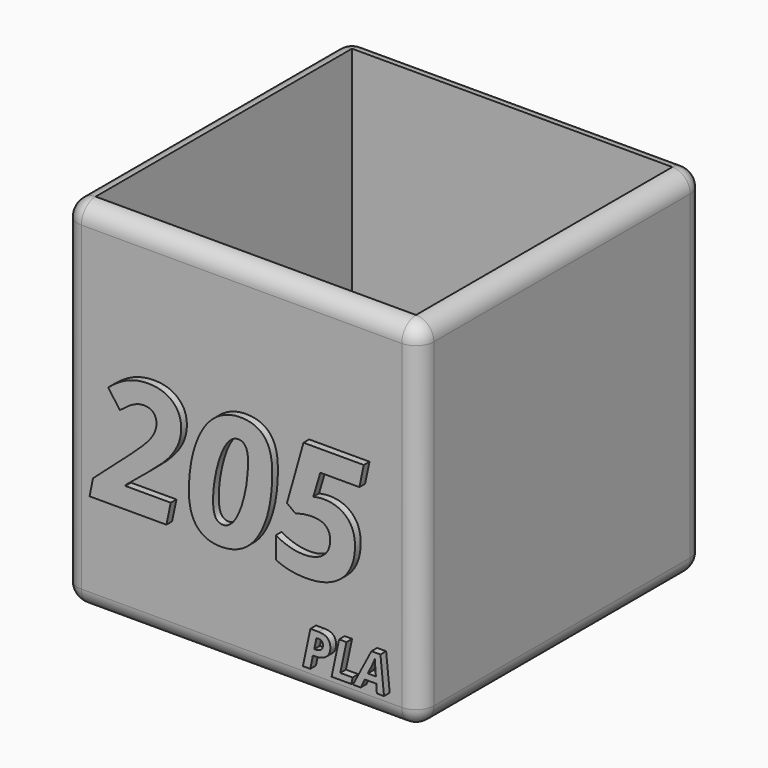
from build123d import *

# Parameters (mm, degrees)
F0_W         = 20
F0_H         = 20
F1_DEPTH     = 20
F2_R         = 1
F3_T         = 1
F4_R         = 0.99999
F7_TEXT_SIZE = 9.189625774
F8_DEPTH     = 0.4
F9_TEXT_SIZE = 2.7777777778
F10_DEPTH    = 0.4


# Not quite as in the source:
# - a fillet or chamfer is up to 0.001 mm smaller than in the source, because OpenCascade refuses the exact size
# - a shell that OpenCascade refuses in one call is made with other operations: the cavity is built on its own and cut out
# - Text() gives the source's letters only with a copy of the font that has no kerning and outlines rounded to 1/6400 em; it was checked with that copy


with BuildPart() as f1:
    # F0 (on Top) → F1 (new body)
    with BuildSketch(Plane.XY):
        Rectangle(F0_W, F0_H)
    extrude(amount=F1_DEPTH)

    # F2
    f2_edges = [f1.edges().sort_by_distance(p)[0] for p in [
        (10, 10, 10),
        (-10, -10, 10),
        (10, -10, 10),
        (-10, 10, 10),
        (10, 0, 0),
        (0, -10, 0),
        (0, 10, 0),
        (-10, 0, 0),
    ]]
    fillet(f2_edges, radius=F2_R)

    # F3: shell of thickness 1, made by hand


with BuildPart() as f3_core1:
    # F3_t2: copy of F1
    add(f1.part)

    # the walls: a layer under each face that stays
    f3_faces = [f3_core1.faces().sort_by_distance(p)[0] for p in [
        (0, -10, 10.5),
        (-10, 0, 10.5),
        (10, 0, 10.5),
        (0, 10, 10.5),
        (0, 0, 0),
    ]]
    thicken(f3_faces, amount=-F3_T, mode=Mode.SUBTRACT)


with BuildPart() as f1_1:
    add(f1.part)

    # what is left inside the walls is the cavity
    f3_cavity = [f3_core1.part.solids().sort_by_distance(p)[0] for p in [
        (-8.99, 0, 13.666667),
    ]]
    add(f3_cavity, mode=Mode.SUBTRACT)

    # F4 (radius 1 in the source; OpenCascade refuses exactly that, so slightly less here)
    f4_edges = [f1_1.edges().sort_by_distance(p)[0] for p in [
        (9.707107, 9.707107, 20),
        (-9.707107, 9.707107, 20),
        (0, -10, 20),
        (0, 10, 20),
        (-9.707107, -9.707107, 20),
        (10, 0, 20),
        (-10, 0, 20),
        (9.707107, -9.707107, 20),
    ]]
    fillet(f4_edges, radius=F4_R)

    # F7 (on face) → F8 (join)
    with BuildSketch(Plane.XZ.offset(10)):
        with Locations((-8, 6)):
            Text('205', F7_TEXT_SIZE, font='Open Sans', font_style=FontStyle.BOLDITALIC, text_align=(TextAlign.LEFT, TextAlign.BOTTOM))
    extrude(amount=F8_DEPTH)

    # F9 (on face) → F10 (join)
    with BuildSketch(Plane.XZ.offset(10)):
        with Locations((3.6918402778, 1.5)):
            Text('PLA', F9_TEXT_SIZE, font='Open Sans', font_style=FontStyle.BOLDITALIC, text_align=(TextAlign.LEFT, TextAlign.BOTTOM))
    extrude(amount=F10_DEPTH)


solid = f1_1.part
